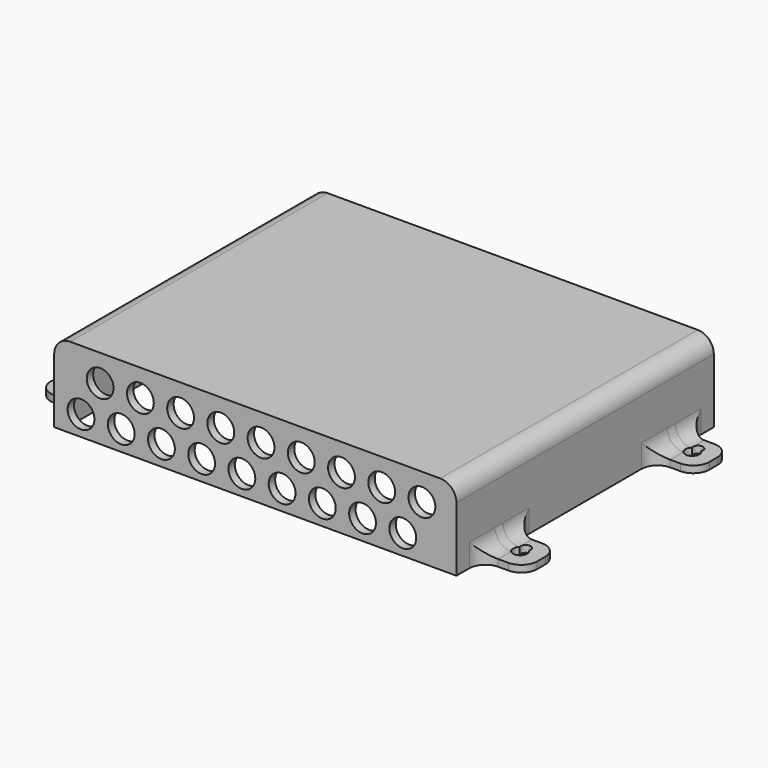
from build123d import *

# Parameters (mm, degrees)
F1_W     = 48
F1_H     = 76
F2_DEPTH = 20
F3_DEPTH = 17
F1_W_2   = 10.5
F1_H_2   = 10.5
F4_DEPTH = 1.7
F5_R     = 3.3333333333
F6_DEPTH = 80.001
F7_R     = 3.99999


# Not quite as in the source:
# - a fillet or chamfer is up to 0.001 mm smaller than in the source, because OpenCascade refuses the exact size
# - a feature names something its author has since deleted; it is built from what else it names


with BuildPart() as f2:
    # F1 (on Top) → F2 (new body)
    with BuildSketch(Plane.XY):
        Polygon((0, 38), (0, 40), (-50, 40), (-50, 32), (-50, 21.5), (-50, -21.5), (-50, -32), (-50, -40), (0, -40), (0, -38), (-48, -38), (-48, 38), align=None)
        Polygon((50, 40), (0, 40), (0, 38), (48, 38), (48, -38), (0, -38), (0, -40), (50, -40), (50, -32), (50, -21.5), (50, 21.5), (50, 32), align=None)
        with Locations((-24, 0)):
            Rectangle(F1_W, F1_H)
        with Locations((24, 0)):
            Rectangle(F1_W, F1_H)
    extrude(amount=F2_DEPTH)

    # F1 (on Top) → F3 (cut)
    with BuildSketch(Plane.XY):
        with Locations((-24, 0)):
            Rectangle(F1_W, F1_H)
        with Locations((24, 0)):
            Rectangle(F1_W, F1_H)
    extrude(amount=F3_DEPTH, mode=Mode.SUBTRACT)

    # F1 (on Top) → F4 (join)
    with BuildSketch(Plane.XY):
        with Locations((-55.25, -26.75)):
            Rectangle(F1_W_2, F1_H_2)
        with BuildLine():
            ThreePointArc((-56.417562217, -25.4464285714), (-55.4769881371, -23.7707822058), (-54, -25))
            ThreePointArc((-54, -25), (-54.0207822058, -25.2269881371), (-54.082437783, -25.4464285714))
            ThreePointArc((-54.082437783, -25.4464285714), (-53.6522306362, -26.0361141127), (-53.5, -26.75))
            ThreePointArc((-53.5, -26.75), (-55.9638858873, -28.3477693638), (-56.417562217, -25.4464285714))
        make_face(mode=Mode.SUBTRACT)
        with Locations((-55.25, 26.75)):
            Rectangle(F1_W_2, F1_H_2)
        with BuildLine():
            ThreePointArc((-56.417562217, 28.0535714286), (-55.4769881371, 29.7292177942), (-54, 28.5))
            ThreePointArc((-54, 28.5), (-54.0207822058, 28.2730118629), (-54.082437783, 28.0535714286))
            ThreePointArc((-54.082437783, 28.0535714286), (-53.6522306362, 27.4638858873), (-53.5, 26.75))
            ThreePointArc((-53.5, 26.75), (-55.9638858873, 25.1522306362), (-56.417562217, 28.0535714286))
        make_face(mode=Mode.SUBTRACT)
        with Locations((55.25, 26.75)):
            Rectangle(F1_W_2, F1_H_2)
        with BuildLine():
            ThreePointArc((56.417562217, 28.0535714286), (56.8477693638, 27.4638858873), (57, 26.75))
            ThreePointArc((57, 26.75), (54.5361141127, 25.1522306362), (54.082437783, 28.0535714286))
            ThreePointArc((54.082437783, 28.0535714286), (55.0230118629, 29.7292177942), (56.5, 28.5))
            ThreePointArc((56.5, 28.5), (56.4792177942, 28.2730118629), (56.417562217, 28.0535714286))
        make_face(mode=Mode.SUBTRACT)
        with Locations((55.25, -26.75)):
            Rectangle(F1_W_2, F1_H_2)
        with BuildLine():
            ThreePointArc((56.417562217, -25.4464285714), (56.8477693638, -26.0361141127), (57, -26.75))
            ThreePointArc((57, -26.75), (54.5361141127, -28.3477693638), (54.082437783, -25.4464285714))
            ThreePointArc((54.082437783, -25.4464285714), (55.0230118629, -23.7707822058), (56.5, -25))
            ThreePointArc((56.5, -25), (56.4792177942, -25.2269881371), (56.417562217, -25.4464285714))
        make_face(mode=Mode.SUBTRACT)
    extrude(amount=F4_DEPTH)

    # F5 (on face) → F6 (cut, through all)
    with BuildSketch(Plane.XZ.offset(40)):
        with Locations((-38.5714285714, 13.3333333333)):
            Circle(F5_R)
        with Locations((-43.3333333333, 5)):
            Circle(F5_R)
        with Locations((-33.3333333333, 5)):
            Circle(F5_R)
        with Locations((-28.5714285714, 13.3333333333)):
            Circle(F5_R)
        with Locations((-23.3333333333, 5)):
            Circle(F5_R)
        with Locations((-18.5714285714, 13.3333333333)):
            Circle(F5_R)
        with Locations((-13.3333333333, 5)):
            Circle(F5_R)
        with Locations((-8.5714285714, 13.3333333333)):
            Circle(F5_R)
        with Locations((-3.3333333333, 5)):
            Circle(F5_R)
        with Locations((1.4285714286, 13.3333333333)):
            Circle(F5_R)
        with Locations((6.6666666667, 5)):
            Circle(F5_R)
        with Locations((11.4285714286, 13.3333333333)):
            Circle(F5_R)
        with Locations((16.6666666667, 5)):
            Circle(F5_R)
        with Locations((21.4285714286, 13.3333333333)):
            Circle(F5_R)
        with Locations((26.6666666667, 5)):
            Circle(F5_R)
        with Locations((31.4285714286, 13.3333333333)):
            Circle(F5_R)
        with Locations((41.4285714286, 13.3333333333)):
            Circle(F5_R)
        with Locations((36.6666666667, 5)):
            Circle(F5_R)
    extrude(amount=-F6_DEPTH, mode=Mode.SUBTRACT)

    # F7 (radius 4 in the source; OpenCascade refuses exactly that, so slightly less here)
    f7_edges = [f2.edges().sort_by_distance(p)[0] for p in [
        (-60.5, 32, 0.85),
        (-60.5, 21.5, 0.85),
        (-50, 21.5, 0.85),
        (-50, -32, 0.85),
        (-60.5, -32, 0.85),
        (-60.5, -21.5, 0.85),
        (-50, 32, 0.85),
        (-50, -21.5, 0.85),
        (-50, 26.75, 1.7),
        (-50, -26.75, 1.7),
        (50, -26.75, 1.7),
        (50, 26.75, 1.7),
        (50, 21.5, 0.85),
        (60.5, 21.5, 0.85),
        (60.5, 32, 0.85),
        (60.5, -21.5, 0.85),
        (60.5, -32, 0.85),
        (50, -32, 0.85),
        (50, -21.5, 0.85),
        (50, 32, 0.85),
        (50, 0, 20),
        (-50, 0, 20),
        (-48, 0, 17),
        (48, 0, 17),
    ]]
    fillet(f7_edges, radius=F7_R)


solid = f2.part
